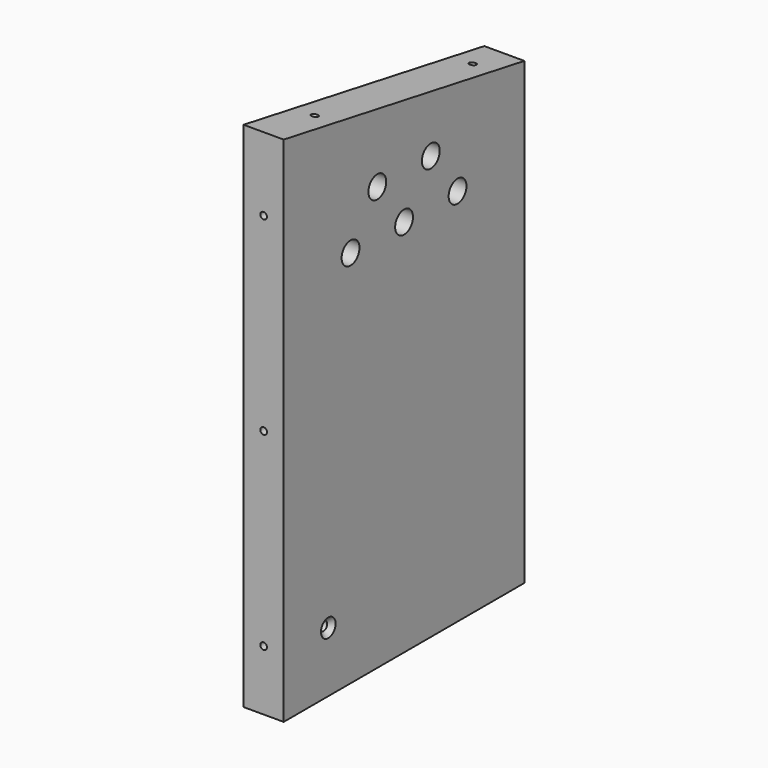
from build123d import *

# Parameters (mm, degrees)
F1_DEPTH       = 18
F2_D           = 10
F3_D           = 10
F5_D           = 4
F5_CSINK_D     = 8.2
F5_CSINK_ANGLE = 90
F7_D           = 3
F7_DEPTH       = 20
F7_TIP         = 0.9012909285
F9_D           = 3
F9_DEPTH       = 20
F9_TIP         = 0.9012909285
F11_D          = 3
F11_DEPTH      = 20
F11_TIP        = 0.9012909285


# Not quite as in the source:
# - a feature names something its author has since deleted; it is built from what else it names


with BuildPart() as f1:
    # F0 (on Right) → F1 (new body)
    with BuildSketch(Plane.YZ):
        Polygon((0, 230), (0, 0), (135, 0), (135, 206.1958576044), align=None)
    extrude(amount=F1_DEPTH)

    # F2 (through all)
    with Locations(Plane(origin=(0, 0, 0), x_dir=(0, 1, 0), z_dir=(-1, 0, 0))):
        with Locations((37.5, -170), (67.5, -170), (97.5, -170)):
            Hole(F2_D / 2)

    # F3 (through all)
    with Locations(Plane(origin=(0, 0, 0), x_dir=(0, 1, 0), z_dir=(-1, 0, 0))):
        with Locations((52.5, -190), (82.5, -190)):
            Hole(F3_D / 2)

    # F5 (through all)
    with Locations(Plane.YZ.offset(18)):
        with Locations((25, 27)):
            CounterSinkHole(F5_D / 2, F5_CSINK_D / 2, counter_sink_angle=F5_CSINK_ANGLE)

    # F7
    with Locations(Plane(origin=(0, 135, 0), x_dir=(-1, 0, 0), z_dir=(0, 1, 0))):
        with Locations((-9, 27), (-9, 106)):
            Hole(F7_D / 2, depth=F7_DEPTH)
            with Locations((0, 0, -(F7_DEPTH + F7_TIP / 2))):  # 118° drill point
                Cone(0, F7_D / 2, F7_TIP, mode=Mode.SUBTRACT)

    # F9
    with Locations(Plane.XZ):
        with Locations((9, 197), (9, 112), (9, 27)):
            Hole(F9_D / 2, depth=F9_DEPTH)
            with Locations((0, 0, -(F9_DEPTH + F9_TIP / 2))):  # 118° drill point
                Cone(0, F9_D / 2, F9_TIP, mode=Mode.SUBTRACT)

    # F11
    with Locations(Plane(origin=(0, 39.3323164825, 223.0646513904), x_dir=(1, 0, 0), z_dir=(0, 0.1736481777, 0.984807753))):
        with Locations((9, -10.8564882588), (9, 79.1435117412)):
            Hole(F11_D / 2, depth=F11_DEPTH)
            with Locations((0, 0, -(F11_DEPTH + F11_TIP / 2))):  # 118° drill point
                Cone(0, F11_D / 2, F11_TIP, mode=Mode.SUBTRACT)


solid = f1.part
